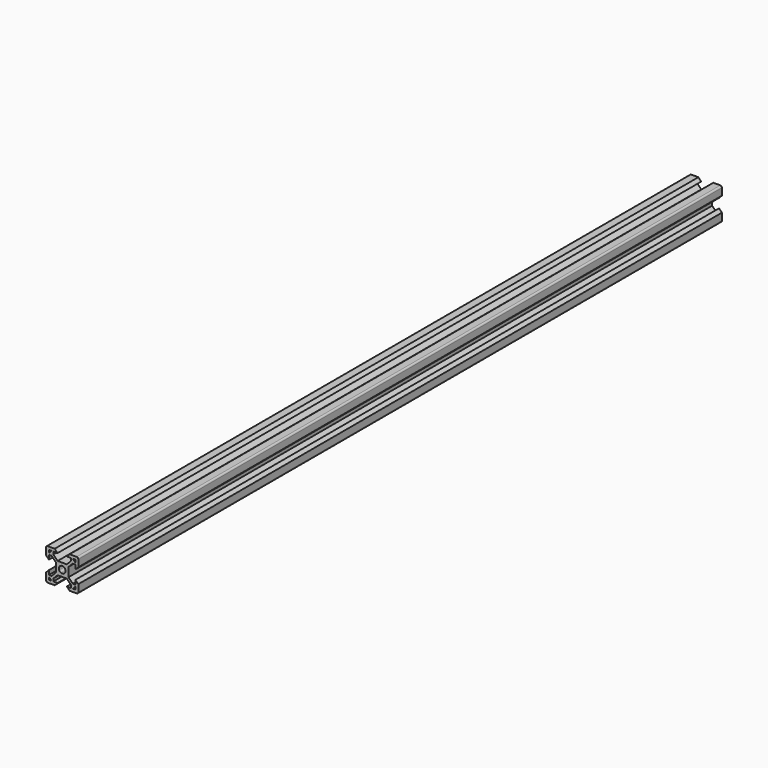
from build123d import *

# Parameters (mm, degrees)
F0_W     = 20
F0_H     = 20
F1_DEPTH = 500
F2_W     = 2.6593398282
F2_H     = 5.68
F2_W_2   = 2.84
F2_H_2   = 2.6593398282
F2_W_3   = 1.64
F2_H_3   = 1.64
F2_H_4   = 1.8
F3_DEPTH = 1000
F5_DEPTH = 100
F6_R     = 1


with BuildPart() as f1:
    # F0 (on Front) → F1 (new body)
    with BuildSketch(Plane.XZ):
        with Locations((10, 10)):
            Rectangle(F0_W, F0_H)
    extrude(amount=F1_DEPTH)

    # F2 (on face) → F3 (cut)
    with BuildSketch(Plane.XZ.offset(500)):
        with BuildLine():
            ThreePointArc((11.9173232366, 9.1433369352), (12.0538231176, 9.5620381277), (12.1, 10))
            ThreePointArc((12.1, 10), (12.0538231176, 10.4379618723), (11.9173232366, 10.8566630648))
            Line((11.9173232366, 10.8566630648), (11.0606601718, 10))
            Line((11.0606601718, 10), (11.9173232366, 9.1433369352))
        make_face()
        with BuildLine():
            Line((11.0606601718, 10), (11.9173232366, 10.8566630648))
            ThreePointArc((11.9173232366, 10.8566630648), (11.4849242405, 11.4849242405), (10.8566630648, 11.9173232366))
            Line((10.8566630648, 11.9173232366), (10, 11.0606601718))
            Line((10, 11.0606601718), (11.0606601718, 10))
        make_face()
        with BuildLine():
            ThreePointArc((11.4849242405, 8.5150757595), (11.7298843892, 8.80941191), (11.9173232366, 9.1433369352))
            Line((11.9173232366, 9.1433369352), (11.0606601718, 10))
            Line((11.0606601718, 10), (10.5303300859, 9.4696699141))
            Line((10.5303300859, 9.4696699141), (11.4849242405, 8.5150757595))
        make_face()
        with BuildLine():
            Line((10, 11.0606601718), (10.8566630648, 11.9173232366))
            ThreePointArc((10.8566630648, 11.9173232366), (10.4379618723, 12.0538231176), (10, 12.1))
            Line((10, 12.1), (10, 11.0606601718))
        make_face()
        Polygon((16.56, 15.4993398282), (13.9006601718, 12.84), (16.56, 12.84), align=None)
        with Locations((15.2303300859, 10)):
            Rectangle(F2_W, F2_H)
        Polygon((10.5303300859, 9.4696699141), (11.0606601718, 10), (10, 11.0606601718), (10, 10), align=None)
        with BuildLine():
            ThreePointArc((10.8566630648, 8.0826767634), (11.19058809, 8.2701156108), (11.4849242405, 8.5150757595))
            Line((11.4849242405, 8.5150757595), (10.5303300859, 9.4696699141))
            Line((10.5303300859, 9.4696699141), (10, 8.9393398282))
            Line((10, 8.9393398282), (10.8566630648, 8.0826767634))
        make_face()
        Polygon((16.56, 7.16), (13.9006601718, 7.16), (16.56, 4.5006601718), align=None)
        with BuildLine():
            Line((10, 11.0606601718), (10, 12.1))
            ThreePointArc((10, 12.1), (9.5620381277, 12.0538231176), (9.1433369352, 11.9173232366))
            Line((9.1433369352, 11.9173232366), (10, 11.0606601718))
        make_face()
        with BuildLine():
            Line((9.4696699141, 10.5303300859), (10, 11.0606601718))
            Line((10, 11.0606601718), (9.1433369352, 11.9173232366))
            ThreePointArc((9.1433369352, 11.9173232366), (8.80941191, 11.7298843892), (8.5150757595, 11.4849242405))
            Line((8.5150757595, 11.4849242405), (9.4696699141, 10.5303300859))
        make_face()
        Polygon((10, 10), (10, 11.0606601718), (9.4696699141, 10.5303300859), align=None)
        Polygon((12.84, 16.56), (12.84, 13.9006601718), (15.4993398282, 16.56), align=None)
        with Locations((11.42, 15.2303300859)):
            Rectangle(F2_W_2, F2_H_2)
        with Locations((17.38, 14.1696699141)):
            Rectangle(F2_W_3, F2_H_2)
        with Locations((17.38, 10)):
            Rectangle(F2_W_3, F2_H)
        Polygon((10, 8.9393398282), (10.5303300859, 9.4696699141), (10, 10), align=None)
        with BuildLine():
            ThreePointArc((10, 7.9), (10.4379618723, 7.9461768824), (10.8566630648, 8.0826767634))
            Line((10.8566630648, 8.0826767634), (10, 8.9393398282))
            Line((10, 8.9393398282), (10, 7.9))
        make_face()
        with Locations((17.38, 5.8303300859)):
            Rectangle(F2_W_3, F2_H_2)
        with Locations((8.58, 15.2303300859)):
            Rectangle(F2_W_2, F2_H_2)
        Polygon((10, 10), (9.4696699141, 10.5303300859), (8.9393398282, 10), (10, 8.9393398282), align=None)
        with BuildLine():
            Line((8.9393398282, 10), (9.4696699141, 10.5303300859))
            Line((9.4696699141, 10.5303300859), (8.5150757595, 11.4849242405))
            ThreePointArc((8.5150757595, 11.4849242405), (8.2701156108, 11.19058809), (8.0826767634, 10.8566630648))
            Line((8.0826767634, 10.8566630648), (8.9393398282, 10))
        make_face()
        with Locations((14.1696699141, 17.38)):
            Rectangle(F2_W, F2_H_3)
        with Locations((11.42, 17.38)):
            Rectangle(F2_W_2, F2_H_3)
        Polygon((20, 12.84), (18.2, 12.84), (18.2, 7.16), (20, 7.16), (20, 10), align=None)
        Polygon((20, 14.64), (18.2, 12.84), (20, 12.84), align=None)
        with BuildLine():
            Line((9.1433369352, 8.0826767634), (10, 8.9393398282))
            Line((10, 8.9393398282), (8.9393398282, 10))
            Line((8.9393398282, 10), (8.0826767634, 9.1433369352))
            ThreePointArc((8.0826767634, 9.1433369352), (8.5150757595, 8.5150757595), (9.1433369352, 8.0826767634))
        make_face()
        with BuildLine():
            Line((10, 7.9), (10, 8.9393398282))
            Line((10, 8.9393398282), (9.1433369352, 8.0826767634))
            ThreePointArc((9.1433369352, 8.0826767634), (9.5620381277, 7.9461768824), (10, 7.9))
        make_face()
        Polygon((15.4993398282, 3.44), (12.84, 6.0993398282), (12.84, 3.44), align=None)
        with Locations((11.42, 4.7696699141)):
            Rectangle(F2_W_2, F2_H_2)
        Polygon((20, 7.16), (18.2, 7.16), (20, 5.36), align=None)
        Polygon((4.5006601718, 16.56), (7.16, 13.9006601718), (7.16, 16.56), align=None)
        with Locations((8.58, 17.38)):
            Rectangle(F2_W_2, F2_H_3)
        with BuildLine():
            Line((8.0826767634, 9.1433369352), (8.9393398282, 10))
            Line((8.9393398282, 10), (8.0826767634, 10.8566630648))
            ThreePointArc((8.0826767634, 10.8566630648), (7.9, 10), (8.0826767634, 9.1433369352))
        make_face()
        Polygon((12.84, 20), (12.84, 18.2), (14.64, 20), align=None)
        with Locations((11.42, 19.1)):
            Rectangle(F2_W_2, F2_H_4)
        with Locations((8.58, 4.7696699141)):
            Rectangle(F2_W_2, F2_H_2)
        with Locations((14.1696699141, 2.62)):
            Rectangle(F2_W, F2_H_3)
        with Locations((11.42, 2.62)):
            Rectangle(F2_W_2, F2_H_3)
        with Locations((5.8303300859, 17.38)):
            Rectangle(F2_W, F2_H_3)
        with Locations((8.58, 19.1)):
            Rectangle(F2_W_2, F2_H_4)
        Polygon((7.16, 3.44), (7.16, 6.0993398282), (4.5006601718, 3.44), align=None)
        with Locations((8.58, 2.62)):
            Rectangle(F2_W_2, F2_H_3)
        with Locations((11.42, 0.9)):
            Rectangle(F2_W_2, F2_H_4)
        Polygon((14.64, 0), (12.84, 1.8), (12.84, 0), align=None)
        Polygon((3.44, 12.84), (6.0993398282, 12.84), (3.44, 15.4993398282), align=None)
        with Locations((4.7696699141, 10)):
            Rectangle(F2_W, F2_H)
        Polygon((5.36, 20), (7.16, 18.2), (7.16, 20), align=None)
        Polygon((3.44, 4.5006601718), (6.0993398282, 7.16), (3.44, 7.16), align=None)
        with Locations((5.8303300859, 2.62)):
            Rectangle(F2_W, F2_H_3)
        with Locations((8.58, 0.9)):
            Rectangle(F2_W_2, F2_H_4)
        with Locations((2.62, 14.1696699141)):
            Rectangle(F2_W_3, F2_H_2)
        with Locations((2.62, 10)):
            Rectangle(F2_W_3, F2_H)
        with Locations((2.62, 5.8303300859)):
            Rectangle(F2_W_3, F2_H_2)
        Polygon((7.16, 0), (7.16, 1.8), (5.36, 0), align=None)
        Polygon((0, 12.84), (1.8, 12.84), (0, 14.64), align=None)
        Polygon((1.8, 7.16), (1.8, 12.84), (0, 12.84), (0, 10), (0, 7.16), align=None)
        Polygon((0, 5.36), (1.8, 7.16), (0, 7.16), align=None)
    extrude(amount=-F3_DEPTH, mode=Mode.SUBTRACT)

    # F4 (on face) → F5 (cut)
    with BuildSketch(Plane.XZ.offset(500)):
        Polygon((3.4306601718, 1.8), (1.8, 3.4306601718), (1.8, 1.8), align=None)
        Polygon((1.8, 18.2), (1.8, 16.5693398282), (3.4306601718, 18.2), align=None)
        Polygon((18.2, 18.2), (16.5693398282, 18.2), (18.2, 16.5693398282), align=None)
        Polygon((18.2, 3.4306601718), (16.5693398282, 1.8), (18.2, 1.8), align=None)
    extrude(amount=-F5_DEPTH, mode=Mode.SUBTRACT)

    # F6
    f6_edges = [f1.edges().sort_by_distance(p)[0] for p in [
        (20, -250, 20),
        (20, -250, 0),
        (0, -250, 20),
        (0, -250, 0),
    ]]
    fillet(f6_edges, radius=F6_R)


solid = f1.part
